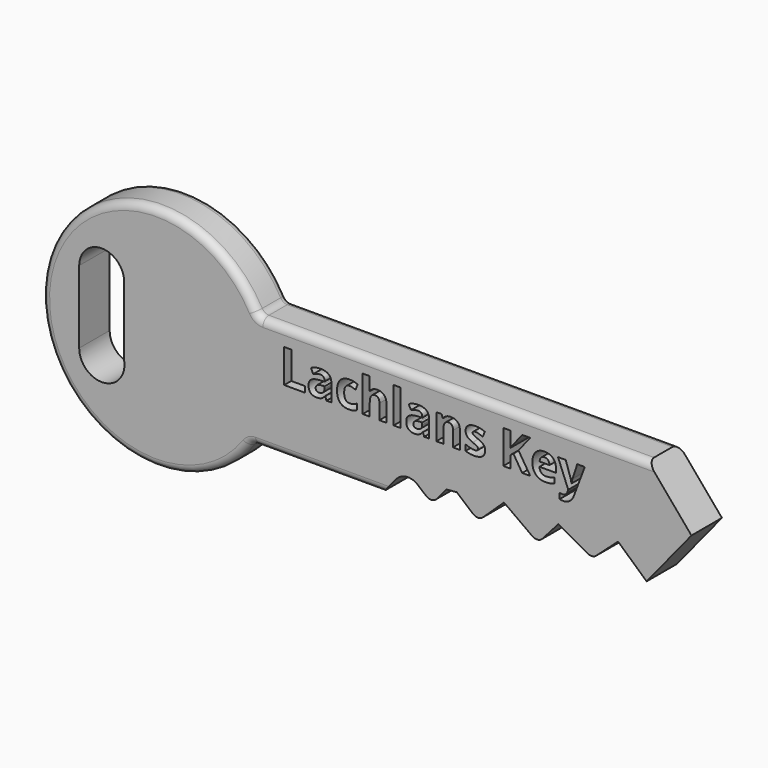
from build123d import *

# Parameters (mm, degrees)
F2_DEPTH     = 5
F3_DEPTH     = 25
F4_TEXT_SIZE = 6.1657032755
F5_DEPTH     = 25
F6_F1_R      = 1
F6_F2_R      = 1
F7_R         = 2
F8_R         = 1
F9_SIZE      = 1


# Not quite as in the source:
# - Text() gives the source's letters only with a copy of the font that has no kerning and outlines rounded to 1/6400 em; it was checked with that copy


with BuildPart() as f2:
    # F0 (on Front) → F2 (new body)
    with BuildSketch(Plane.XZ):
        with BuildLine():
            Line((64.5457310282, 6.7468107205), (13.3970349369, 6.7468107205))
            ThreePointArc((13.3970349369, 6.7468107205), (-14.9747372431, 0.8701979658), (12.5253689254, -8.2531892795))
            Line((12.5253689254, -8.2531892795), (29.6865933297, -8.2531892795))
            Line((29.6865933297, -8.2531892795), (32.8078016303, -4.5467514458))
            Line((32.8078016303, -4.5467514458), (36.1955383821, -7.3995801035))
            Line((36.1955383821, -7.3995801035), (38.6917800067, -4.3684271962))
            Line((38.6917800067, -4.3684271962), (42.257845938, -7.3995801035))
            Line((42.257845938, -7.3995801035), (45.6456049161, -4.1901237255))
            Line((45.6456049161, -4.1901237255), (50.1031812357, -7.3995801035))
            Line((50.1031812357, -7.3995801035), (52.7777298136, -4.3684271962))
            Line((52.7777298136, -4.3684271962), (57.2353096158, -6.8646709974))
            Line((57.2353096158, -6.8646709974), (60.6230685938, -3.8335176548))
            Line((60.6230685938, -3.8335176548), (64.3674345133, -7.2212770682))
            Line((64.3674345133, -7.2212770682), (70.2514420811, 0))
            Line((70.2514420811, 0), (64.5457310282, 6.7468107205))
        make_face()
    extrude(amount=F2_DEPTH)

    # F1 (on Front) → F3 (cut)
    with BuildSketch(Plane.XZ):
        with BuildLine():
            ThreePointArc((-4.1959956288, 5.0542671233), (-7.1522644721, 8.0105359666), (-10.1085333154, 5.0542671233))
            Line((-10.1085333154, 5.0542671233), (-10.1085333154, -4.4820858166))
            ThreePointArc((-10.1085333154, -4.4820858166), (-6.9488360437, -7.4445007507), (-4.1959956288, -4.1006319225))
            Line((-4.1959956288, -4.1006319225), (-4.1959956288, 5.0542671233))
        make_face()
    extrude(amount=F3_DEPTH, mode=Mode.SUBTRACT)

    # F4 (on Front) → F5 (cut)
    with BuildSketch(Plane.XZ):
        with Locations((16.2478001602, 0)):
            Text('Lachlans Key', F4_TEXT_SIZE, font='Open Sans', font_style=FontStyle.BOLD, text_align=(TextAlign.LEFT, TextAlign.BOTTOM))
    extrude(amount=F5_DEPTH, mode=Mode.SUBTRACT)

    # F6: fillet of radius 1 on 7 edges, made by hand

    # F6_f1
    f6_f1_edges = [f2.edges().sort_by_distance(p)[0] for p in [
        (12.5253689254, -2.5, -8.2531892795),
        (13.3970349369, -2.5, 6.7468107205),
    ]]
    fillet(f6_f1_edges, radius=F6_F1_R)

    # F6_f2
    f6_f2_edges = [f2.edges().sort_by_distance(p)[0] for p in [
        (29.6865933297, -2.5, -8.2531892795),
        (21.3697522143, 0, -8.2531892795),
        (21.3697522143, -5, -8.2531892795),
        (-14.9767989319, 0, 0.833962681),
        (-14.9767989319, -5, 0.833962681),
        (13.491682446, -5, 6.8853655191),
        (12.5937402865, -5, -8.3648412818),
        (13.491682446, 0, 6.8853655191),
        (12.5937402865, 0, -8.3648412818),
    ]]
    fillet(f6_f2_edges, radius=F6_F2_R)

    # F7
    f7_edges = [f2.edges().sort_by_distance(p)[0] for p in [
        (32.807802, -2.5, -4.546751),
    ]]
    fillet(f7_edges, radius=F7_R)

    # F8
    f8_edges = [f2.edges().sort_by_distance(p)[0] for p in [
        (36.195538, -2.5, -7.39958),
        (42.257846, -2.5, -7.39958),
        (50.103181, -2.5, -7.39958),
        (57.23531, -2.5, -6.864671),
    ]]
    fillet(f8_edges, radius=F8_R)

    # F9
    f9_edges = [f2.edges().sort_by_distance(p)[0] for p in [
        (38.69178, -2.5, -4.368427),
    ]]
    chamfer(f9_edges, length=F9_SIZE)


solid = f2.part
